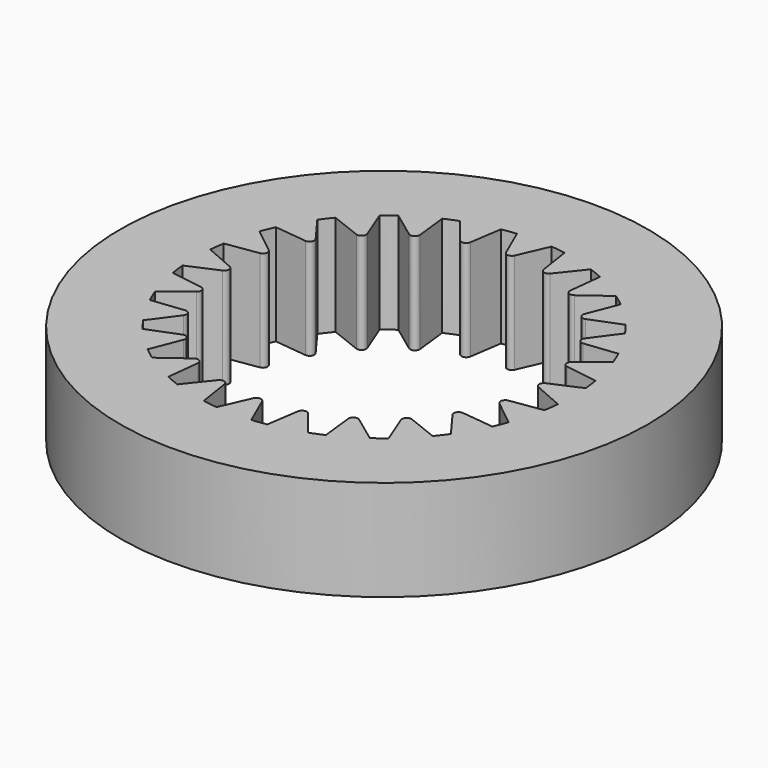
from build123d import *

# Parameters (mm, degrees)
F0_R            = 11.9016009371
F1_DEPTH        = 6.35
F3_DEPTH        = 6.35
F4_R            = 16.6641009371
F5_DEPTH        = 6.35
F5_COPIES_COUNT = 24
F6_DEPTH        = 6.35


# Not quite as in the source:
# - a pattern or mirror of a feature is missing from the dataset's text; its kind, count and spacing are read off the source's solid


with BuildPart() as f1:
    # F0 (on Top) → F1 (new body)
    with BuildSketch(Plane.XY):
        Circle(F0_R)
    extrude(amount=F1_DEPTH)

    # F2 (on face) → F3 (cut, through all)
    with BuildSketch(Plane.XY.offset(6.35)):
        with BuildLine():
            Line((0.272684092, 9.968449005), (1.0946616999, 11.8511527131))
            ThreePointArc((1.0946616999, 11.8511527131), (0, 11.9016009371), (-1.0946616999, 11.8511527131))
            Line((-1.0946616999, 11.8511527131), (-0.272684092, 9.968449005))
            ThreePointArc((-0.272684092, 9.968449005), (0, 9.7899612874), (0.272684092, 9.968449005))
        make_face()
    extrude(amount=-F3_DEPTH, mode=Mode.SUBTRACT)



with BuildPart() as f5:
    # F4 (on face) → F5 (new body)
    with BuildSketch(Plane.XY.offset(6.35)):
        Circle(F4_R)
        with BuildLine():
            Line((-1.0946616999, 11.8511527131), (-0.272684092, 9.968449005))
            ThreePointArc((-0.272684092, 9.968449005), (0, 9.7899612874), (0.272684092, 9.968449005))
            Line((0.272684092, 9.968449005), (1.0946616999, 11.8511527131))
            ThreePointArc((1.0946616999, 11.8511527131), (0, -11.9016009371), (-1.0946616999, 11.8511527131))
        make_face(mode=Mode.SUBTRACT)
    extrude(amount=F5_DEPTH)


with BuildPart() as f1_1:
    add(f1.part)

    add(f5.part)  # F5_copies merges F5
    # F5_copies: F5 ×24 about axis
    f5_copies_axis = Axis((0, 0, 0), (0, 0, 1))
    for i in range(1, F5_COPIES_COUNT):
        add(f5.part.rotate(f5_copies_axis, i * 360 / F5_COPIES_COUNT))

    # F6 (cut, through all): a face of the model
    f6_faces = [f1_1.faces().sort_by_distance(p)[0] for p in [
        (0, -0.0681451869, 0),
    ]]
    extrude(f6_faces, amount=-F6_DEPTH, mode=Mode.SUBTRACT)


solid = f1_1.part
